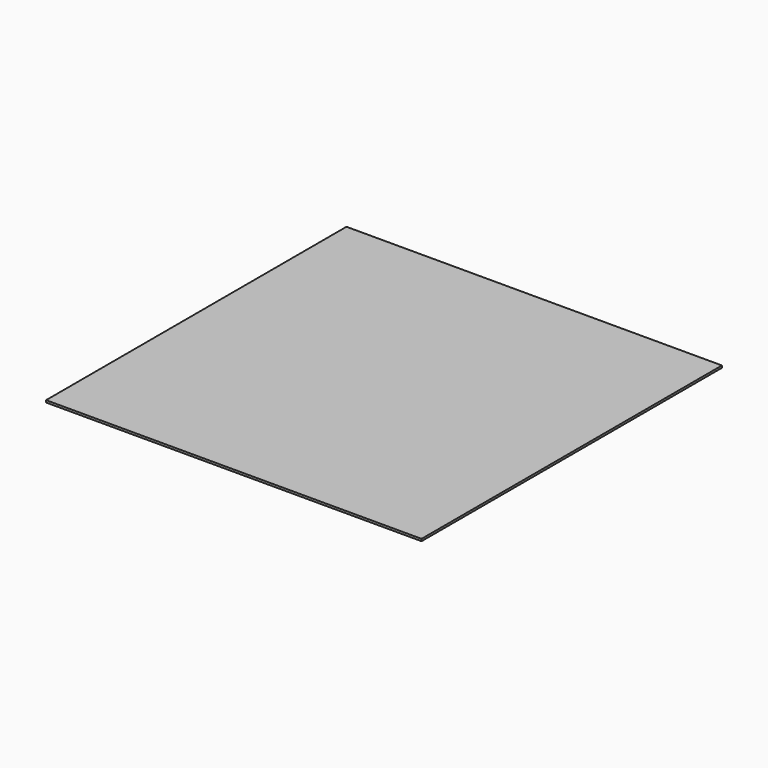
from build123d import *

# Parameters (mm, degrees)
F0_W     = 279.4
F0_H     = 279.4
F1_DEPTH = 1.5875


# Not quite as in the source:
# - a length typed as a fraction of an inch, garbled in the dataset ("3 / 203.2 mm" for 3/8 in), is restored


with BuildPart() as f1:
    # F0 (on Top) → F1 (new body)
    with BuildSketch(Plane.XY):
        with Locations((-7.2494596243, 31.2117603402)):
            Rectangle(F0_W, F0_H)
    extrude(amount=F1_DEPTH)


solid = f1.part
